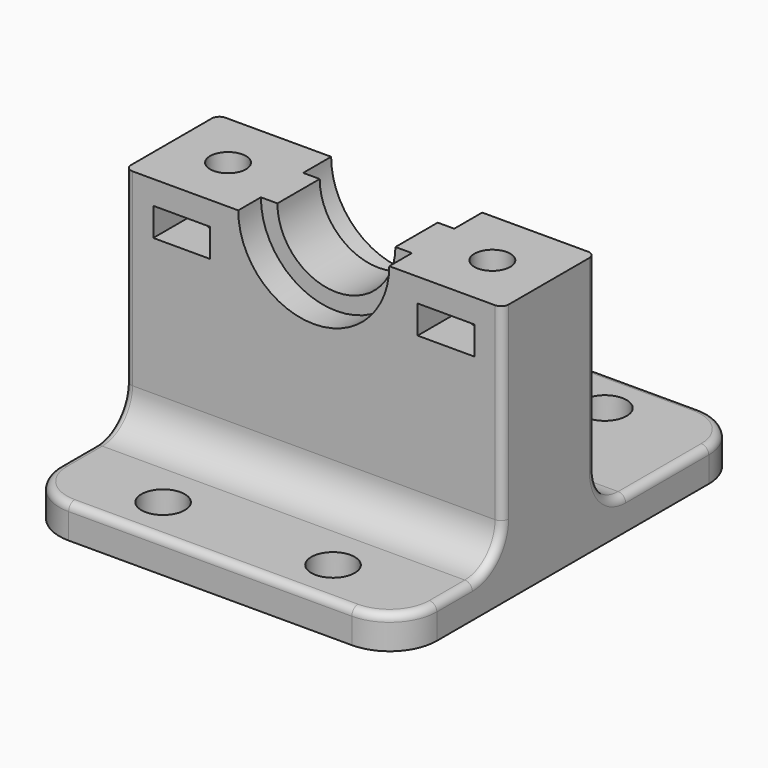
from build123d import *

# Parameters (mm, degrees)
F0_W          = 40
F0_H          = 46
F0_R          = 2.3
F1_DEPTH      = 3.5
F2_W          = 40
F2_H          = 12.3
F3_DEPTH      = 24
F4_R          = 4
F6_DEPTH      = 25
F7_R          = 5
F8_R          = 1.9
F9_DEPTH      = 10
F10_W         = 6
F10_H         = 3
F11_DEPTH     = 25
F13_DEPTH     = 3
F15_DEPTH     = 3.7
F16_R         = 0.8
F17_TEXT_SIZE = 6.9444444444
F18_DEPTH     = 0.6


# Not quite as in the source:
# - Text() gives the source's letters only with a copy of the font that has no kerning and outlines rounded to 1/6400 em; it was checked with that copy


with BuildPart() as f1:
    # F0 (on Top) → F1 (new body)
    with BuildSketch(Plane.XY):
        with Locations((-4.706298545, -3.4629701003)):
            Rectangle(F0_W, F0_H)
        with Locations((-13.706298545, -21.4629701003)):
            Circle(F0_R, mode=Mode.SUBTRACT)
        with Locations((4.293701455, -21.4629701003)):
            Circle(F0_R, mode=Mode.SUBTRACT)
        with Locations((-13.706298545, 14.5370298997)):
            Circle(F0_R, mode=Mode.SUBTRACT)
        with Locations((4.293701455, 14.5370298997)):
            Circle(F0_R, mode=Mode.SUBTRACT)
    extrude(amount=F1_DEPTH)

    # F2 (on face) → F3 (join)
    with BuildSketch(Plane.XY.offset(3.5)):
        with Locations((-4.706298545, -6.6129701003)):
            Rectangle(F2_W, F2_H)
    extrude(amount=F3_DEPTH)

    # F4
    f4_edges = [f1.edges().sort_by_distance(p)[0] for p in [
        (-4.706299, -12.76297, 3.5),
        (-4.706299, -0.46297, 3.5),
    ]]
    fillet(f4_edges, radius=F4_R)

    # F5 (on face) → F6 (cut)
    with BuildSketch(Plane(origin=(0, -0.4629701003, 0), x_dir=(-1, 0, 0), z_dir=(0, 1, 0))):
        with BuildLine():
            ThreePointArc((-1.543701455, 27.5), (4.706298545, 21.25), (10.956298545, 27.5))
            Line((10.956298545, 27.5), (-1.543701455, 27.5))
        make_face()
    extrude(amount=-F6_DEPTH, mode=Mode.SUBTRACT)

    # F7
    f7_edges = [f1.edges().sort_by_distance(p)[0] for p in [
        (15.293701, 19.53703, 1.75),
        (-24.706299, 19.53703, 1.75),
        (15.293701, -26.46297, 1.75),
        (-24.706299, -26.46297, 1.75),
    ]]
    fillet(f7_edges, radius=F7_R)

    # F8 (on face) → F9 (cut)
    with BuildSketch(Plane.XY.offset(27.5)):
        with Locations((-18.706298545, -6.6129701003)):
            Circle(F8_R)
        with Locations((9.293701455, -6.6129701003)):
            Circle(F8_R)
    extrude(amount=-F9_DEPTH, mode=Mode.SUBTRACT)

    # F10 (on face) → F11 (cut)
    with BuildSketch(Plane(origin=(0, -0.4629701003, 0), x_dir=(-1, 0, 0), z_dir=(0, 1, 0))):
        with Locations((18.706298545, 23.5)):
            Rectangle(F10_W, F10_H)
        with Locations((-9.293701455, 23.5)):
            Rectangle(F10_W, F10_H)
    extrude(amount=-F11_DEPTH, mode=Mode.SUBTRACT)

    # F12 (on face) → F13 (cut)
    with BuildSketch(Plane.XZ.offset(12.7629701003)):
        with BuildLine():
            ThreePointArc((-12.706298545, 27.5), (-4.706298545, 19.5), (3.293701455, 27.5))
            Line((3.293701455, 27.5), (1.543701455, 27.5))
            ThreePointArc((1.543701455, 27.5), (-4.706298545, 21.25), (-10.956298545, 27.5))
            Line((-10.956298545, 27.5), (-12.706298545, 27.5))
        make_face()
    extrude(amount=-F13_DEPTH, mode=Mode.SUBTRACT)

    # F14 (on face) → F15 (cut)
    with BuildSketch(Plane(origin=(0, -0.4629701003, 0), x_dir=(-1, 0, 0), z_dir=(0, 1, 0))):
        with BuildLine():
            ThreePointArc((-3.293701455, 27.5), (4.706298545, 19.5), (12.706298545, 27.5))
            Line((12.706298545, 27.5), (10.956298545, 27.5))
            ThreePointArc((10.956298545, 27.5), (4.706298545, 21.25), (-1.543701455, 27.5))
            Line((-1.543701455, 27.5), (-3.293701455, 27.5))
        make_face()
    extrude(amount=-F15_DEPTH, mode=Mode.SUBTRACT)

    # F16
    f16_edges = [f1.edges().sort_by_distance(p)[0] for p in [
        (-24.706299, -12.76297, 17.5),
        (15.293701, -12.76297, 17.5),
        (15.293701, -0.46297, 17.5),
        (-24.706299, -0.46297, 17.5),
        (15.293701, -19.11297, 3.5),
        (15.293701, -13.934543, 4.671573),
        (15.293701, 9.03703, 3.5),
        (15.293701, 0.708603, 4.671573),
        (-24.706299, -19.11297, 3.5),
        (-23.241832, -24.998504, 3.5),
        (-4.706299, -26.46297, 3.5),
        (13.829235, -24.998504, 3.5),
        (-24.706299, -13.934543, 4.671573),
        (13.829235, 18.072564, 3.5),
        (-24.706299, 9.03703, 3.5),
        (-23.241832, 18.072564, 3.5),
        (-4.706299, 19.53703, 3.5),
        (-24.706299, 0.708603, 4.671573),
    ]]
    fillet(f16_edges, radius=F16_R)

    # F17 (on face) → F18 (join)
    with BuildSketch(Plane.XY.offset(3.5)):
        with Locations((-9.1648488922, 6.7370298997)):
            Text('RT', F17_TEXT_SIZE, font='Open Sans', font_style=FontStyle.BOLD, text_align=(TextAlign.LEFT, TextAlign.BOTTOM))
    extrude(amount=F18_DEPTH)


solid = f1.part
